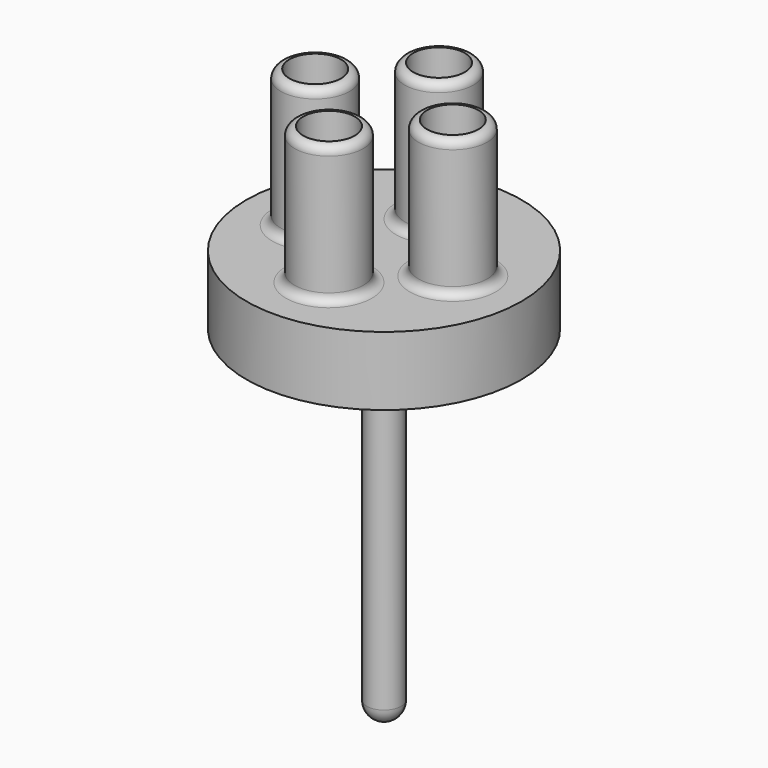
from build123d import *

# Parameters (mm, degrees)
F0_R            = 50.8
F1_DEPTH        = 25.4
F2_R            = 12.7
F3_DEPTH        = 50.8
F3_COPIES_COUNT = 4
F4_R            = 9.525
F5_DEPTH        = 76.201
F5_COPIES_COUNT = 4
F6_R            = 3.17499
F7_R            = 6.35
F8_DEPTH        = 127
F9_R            = 6.35


# Not quite as in the source:
# - a fillet or chamfer is up to 0.001 mm smaller than in the source, because OpenCascade refuses the exact size
# - a pattern or mirror of a feature is missing from the dataset's text; its kind, count and spacing are read off the source's solid


with BuildPart() as f1:
    # F0 (on Top) → F1 (new body)
    with BuildSketch(Plane.XY):
        Circle(F0_R)
    extrude(amount=F1_DEPTH)

    # F2 (on face) → F3 (join)
    with BuildSketch(Plane.XY.offset(25.4)):
        with Locations((0, 25.4)):
            Circle(F2_R)
    f3 = extrude(amount=F3_DEPTH)

    # F3_copies: F3 ×4 about axis
    f3_copies_axis = Axis((0, 0, 0), (0, 0, 1))
    for i in range(1, F3_COPIES_COUNT):
        add(f3.rotate(f3_copies_axis, i * 360 / F3_COPIES_COUNT))

    # F4 (on face) → F5 (cut, through all)
    with BuildSketch(Plane.XY.offset(76.2)):
        with Locations((0, 25.4)):
            Circle(F4_R)
    f5 = extrude(amount=-F5_DEPTH, mode=Mode.SUBTRACT)

    # F5_copies: F5 ×4 about axis
    f5_copies_axis = Axis((0, 0, 0), (0, 0, 1))
    for i in range(1, F5_COPIES_COUNT):
        add(f5.rotate(f5_copies_axis, i * 360 / F5_COPIES_COUNT), mode=Mode.SUBTRACT)

    # F6 (radius 3.175 in the source; OpenCascade refuses exactly that, so slightly less here)
    f6_edges = [f1.edges().sort_by_distance(p)[0] for p in [
        (-12.7, 25.4, 76.2),
        (-12.7, 25.4, 25.4),
        (12.7, -25.4, 25.4),
        (-25.4, -12.7, 25.4),
        (25.4, 12.7, 25.4),
        (12.7, -25.4, 76.2),
        (-25.4, -12.7, 76.2),
        (25.4, 12.7, 76.2),
    ]]
    fillet(f6_edges, radius=F6_R)

    # F7 (on face) → F8 (join)
    with BuildSketch(Plane(origin=(0, 0, 0), x_dir=(1, 0, 0), z_dir=(0, 0, -1))):
        Circle(F7_R)
    extrude(amount=F8_DEPTH)

    # F9
    f9_edges = [f1.edges().sort_by_distance(p)[0] for p in [
        (-6.35, 0, -127),
    ]]
    fillet(f9_edges, radius=F9_R)


solid = f1.part
